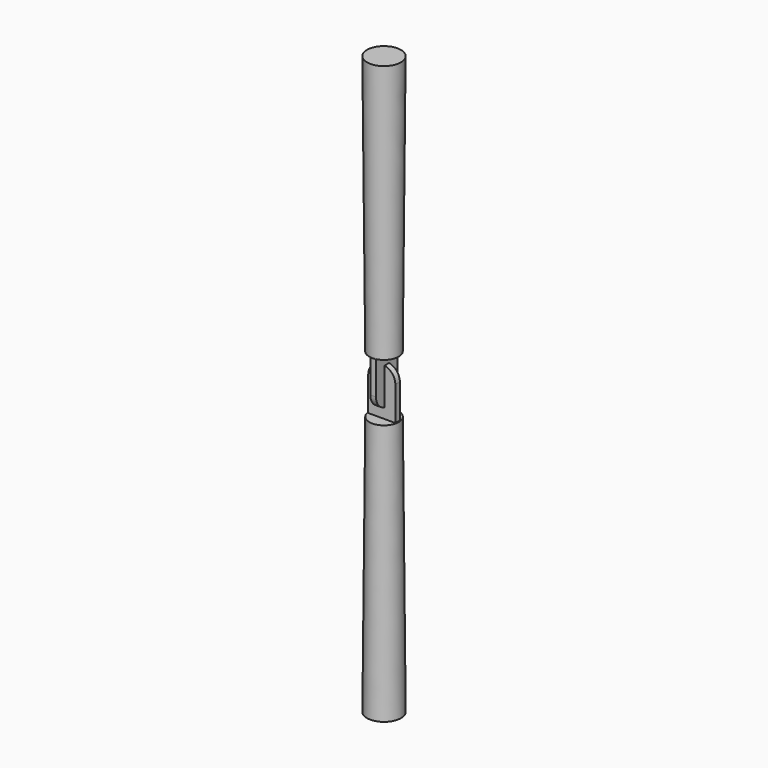
from build123d import *

# Parameters (mm, degrees)
F0_W     = 6
F0_H     = 15
F2_DEPTH = 1.25
F3_W     = 6
F3_H     = 15
F5_DEPTH = 1.25


# Not quite as in the source:
# - a feature names something its author has since deleted; it is built from what else it names


with BuildPart() as f1:
    # F0 (on Front) → F1 (revolve)
    with BuildSketch(Plane.XZ):
        Polygon((0, -115), (0, 0), (-6, 0), (-6.5, 0), (-7.5, -115), align=None)
    revolve(axis=Axis((0, 0, -57.5), (0, 0, 1)))

    # F0 (on Front) → F2 (join, symmetric)
    with BuildSketch(Plane.XZ):
        with Locations((-3, 7.5)):
            Rectangle(F0_W, F0_H)
        with Locations((3, 7.5)):
            Rectangle(F0_W, F0_H)
        with BuildLine():
            Line((-6, 15), (0, 15))
            Line((0, 15), (6, 15))
            ThreePointArc((6, 15), (0, 21), (-6, 15))
        make_face()
    extrude(amount=F2_DEPTH, both=True)


with BuildPart() as f4:
    # F3 (on Right) → F4 (revolve)
    with BuildSketch(Plane.YZ):
        Polygon((-6, 25.5), (-0.0391304348, 25.5), (-0.0391304348, 140.5), (-7.5391304348, 140.5), (-6.5391304348, 25.5), align=None)
    revolve(axis=Axis((0, -0.0391304348, 83), (0, 0, 1)))


with BuildPart() as f5:
    # F3 (on Right) → F5 (new body, symmetric)
    with BuildSketch(Plane.YZ):
        Polygon((0, 10.5), (0, 25.5), (-0.0391304348, 25.5), (-6, 25.5), (-6, 10.5), align=None)
        with Locations((3, 18)):
            Rectangle(F3_W, F3_H)
        with BuildLine():
            Line((6, 10.5), (0, 10.5))
            Line((0, 10.5), (-6, 10.5))
            ThreePointArc((-6, 10.5), (-4.2426406871, 6.2573593129), (0, 4.5))
            ThreePointArc((0, 4.5), (4.2426406871, 6.2573593129), (6, 10.5))
        make_face()
    extrude(amount=F5_DEPTH, both=True)


solid = Compound([f1.part, f4.part, f5.part])
